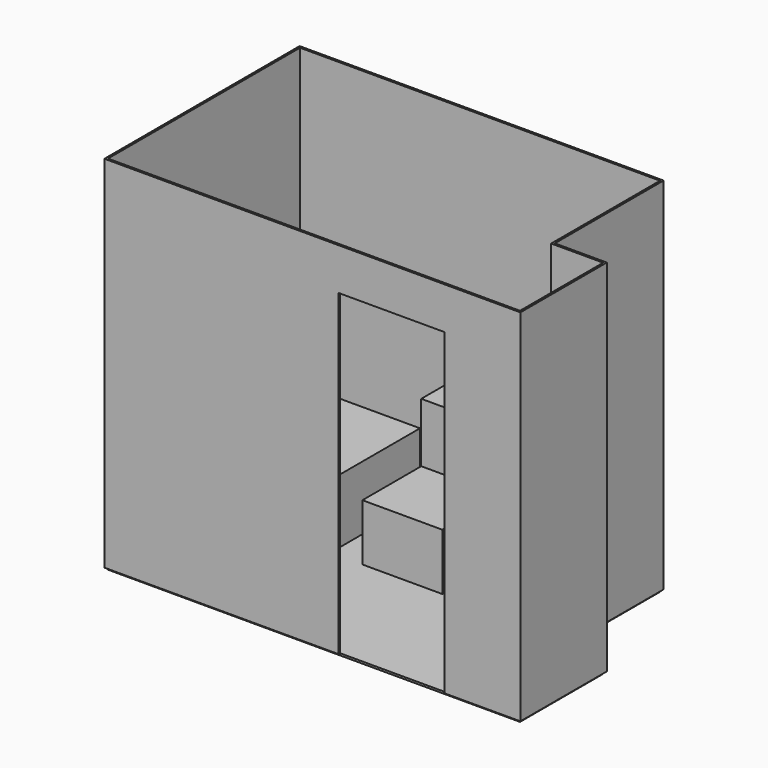
from build123d import *

# Parameters (mm, degrees)
F1_DEPTH  = 12.7
F3_DEPTH  = 2286
F4_W      = 673.1
F4_H      = 2019.3
F5_DEPTH  = 25.4
F6_W      = 762
F6_H      = 1524
F8_DEPTH  = 406.4
F9_W      = 508
F9_H      = 736.6
F10_DEPTH = 711.2
F9_W_2    = 533.4
F9_H_2    = 609.6
F11_DEPTH = 254
F12_W     = 467.0596377373
F12_H     = 377.0357254505
F13_DEPTH = 762


with BuildPart() as f1:
    # F0 (on Top) → F1 (new body)
    with BuildSketch(Plane.XY):
        Polygon((-1143, -762), (1143, -762), (1473.2, -762), (1473.2, -101.6), (1143, -101.6), (1143, 762), (-1143, 762), align=None)
    extrude(amount=-F1_DEPTH)


with BuildPart() as f3:
    # F2 (on face) → F3 (new body)
    with BuildSketch(Plane.XY):
        Polygon((-1155.7, -774.7), (1485.9, -774.7), (1485.9, -88.9), (1155.7, -88.9), (1155.7, 774.7), (-1155.7, 774.7), align=None)
        Polygon((1473.2, -762), (-1143, -762), (-1143, 762), (1143, 762), (1143, -101.6), (1473.2, -101.6), align=None, mode=Mode.SUBTRACT)
    extrude(amount=F3_DEPTH)

    # F4 (on face) → F5 (cut)
    with BuildSketch(Plane.XZ.offset(774.7)):
        with Locations((666.75, 1009.65)):
            Rectangle(F4_W, F4_H)
    extrude(amount=-F5_DEPTH, mode=Mode.SUBTRACT)

    # F9 (on face) → F11 (join)
    with BuildSketch(Plane.XZ.offset(-762)):
        with Locations((800.1, 457.2)):
            Rectangle(F9_W_2, F9_H_2)
    extrude(amount=F11_DEPTH)


with BuildPart() as f8:
    # F6 (on face) → F8 (new body)
    with BuildSketch(Plane.XY):
        with Locations((-762, 0)):
            Rectangle(F6_W, F6_H)
    extrude(amount=F8_DEPTH)


with BuildPart() as f10:
    # F9 (on face) → F10 (new body)
    with BuildSketch(Plane.XZ.offset(-762)):
        with Locations((76.2, 368.3)):
            Rectangle(F9_W, F9_H)
    extrude(amount=F10_DEPTH)

    # F12 (on face) → F13 (cut)
    with BuildSketch(Plane.YZ.offset(330.2)):
        with Locations((284.3298188686, 548.0821372747)):
            Rectangle(F12_W, F12_H)
    extrude(amount=-F13_DEPTH, mode=Mode.SUBTRACT)


solid = Compound([f1.part, f3.part, f8.part, f10.part])
